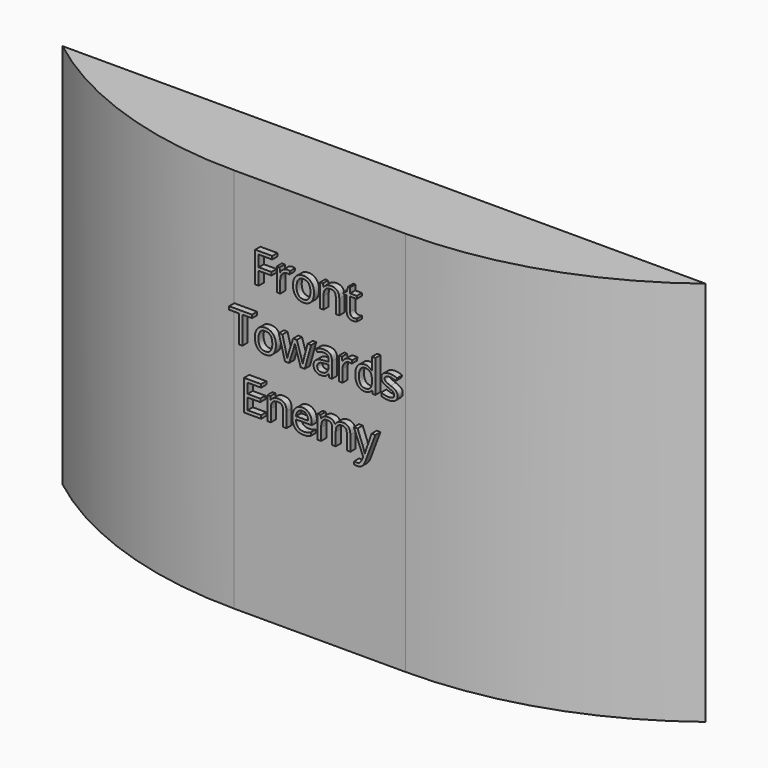
from build123d import *

# Parameters (mm, degrees)
F0_W          = 200
F0_H          = 120
F1_DEPTH      = 25
F2_T1_DEPTH   = 486.5719574654
F3_T          = -2.5
F4_TEXT_SIZE  = 13.3152375507
F5_DEPTH      = 2
F5_DEPTH_BACK = 2


# Not quite as in the source:
# - a fillet or chamfer that OpenCascade refuses, or shapes differently, is made with other operations: its cross-section is extruded or revolved along the edge and cut away or added
# - Text() gives the source's letters only with a copy of the font that has no kerning and outlines rounded to 1/6400 em; it was checked with that copy


with BuildPart() as f1:
    # F0 (on Front) → F1 (new body)
    with BuildSketch(Plane.XZ):
        with Locations((4.3428316712, -24.1487745444)):
            Rectangle(F0_W, F0_H)
    extrude(amount=F1_DEPTH)

    # F2: fillet of radius 120 on 2 edges, made by hand

    # F2_s2 → F2_t1 (cut)
    with BuildSketch(Plane.XY.offset(-267.4347532771)):
        with BuildLine():
            ThreePointArc((-95.6571683288, 0), (-61.0726102978, -18.578166916), (-22.3427768357, -25))
            Line((-22.3427768357, -25), (-95.6571683288, -25))
            Line((-95.6571683288, -25), (-95.6571683288, 0))
        make_face()
        with BuildLine():
            ThreePointArc((104.3428316712, 0), (69.7582736402, -18.578166916), (31.0284401782, -25))
            Line((31.0284401782, -25), (104.3428316712, -25))
            Line((104.3428316712, -25), (104.3428316712, 0))
        make_face()
    extrude(amount=F2_T1_DEPTH, mode=Mode.SUBTRACT)

    # F3
    f3_openings = [f1.faces().sort_by_distance(p)[0] for p in [
        (4.342832, 0, -24.148775),
    ]]
    offset(amount=F3_T, openings=f3_openings)

    # F4 (on face) → F5 (join, two sides)
    with BuildSketch(Plane.XZ.offset(25)) as f5_sk:
        with Locations((-15.423014321, 8.1009533358)):
            Text('Front', F4_TEXT_SIZE, font='Open Sans', text_align=(TextAlign.LEFT, TextAlign.BOTTOM))
        with Locations((-22.3427768357, -10.0077697332)):
            Text('Towards', F4_TEXT_SIZE, font='Open Sans', text_align=(TextAlign.LEFT, TextAlign.BOTTOM))
        with Locations((-18.8828955784, -28.1164928022)):
            Text('Enemy', F4_TEXT_SIZE, font='Open Sans', text_align=(TextAlign.LEFT, TextAlign.BOTTOM))
    extrude(amount=F5_DEPTH)
    extrude(f5_sk.sketch, amount=-F5_DEPTH_BACK)


solid = f1.part
